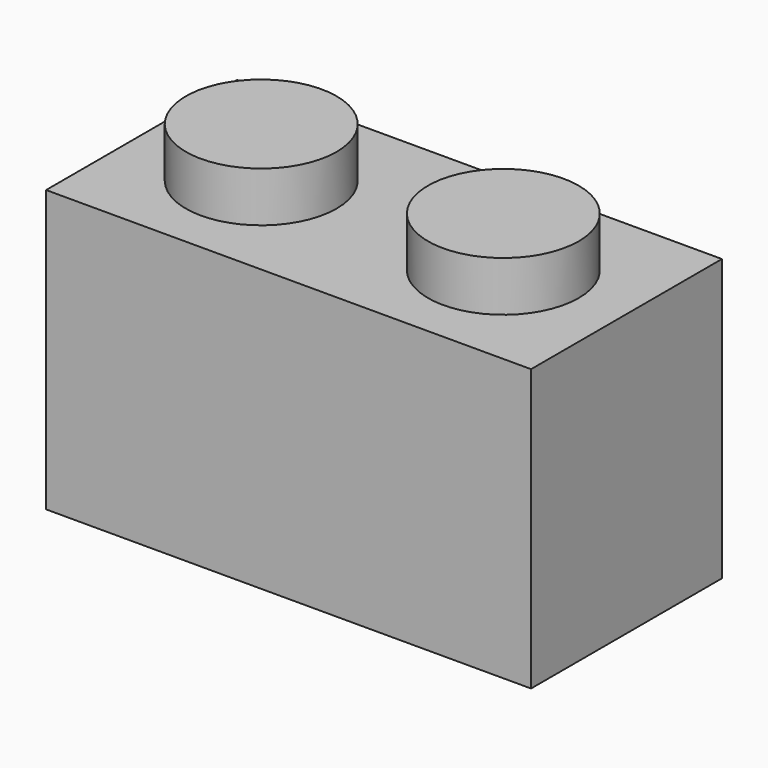
from build123d import *

# Parameters (mm, degrees)
F0_W      = 15.7734
F0_H      = 7.7597
F1_DEPTH  = 9.144
F2_R      = 2.4511
F3_DEPTH  = 1.6256
F5_W      = 13.0048
F5_H      = 4.953
F6_DEPTH  = 8.128
F7_R      = 1.5455831521
F8_DEPTH  = 8.128
F10_R     = 1.4732
F11_DEPTH = 8.128


# Not quite as in the source:
# - a feature names something its author has since deleted; it is built from what else it names


with BuildPart() as f1:
    # F0 (on Top) → F1 (new body)
    with BuildSketch(Plane.XY):
        with Locations((-0.3538653118, -22.1200450051)):
            Rectangle(F0_W, F0_H)
    extrude(amount=F1_DEPTH)

    # F2 (on face) → F3 (join)
    with BuildSketch(Plane.XY.offset(9.144)):
        with Locations((-4.2908653118, -22.1898950051)):
            Circle(F2_R)
        with Locations((3.5837523812, -22.1898950051)):
            Circle(F2_R)
    extrude(amount=F3_DEPTH)

    # F5 (on face) → F6 (cut)
    with BuildSketch(Plane(origin=(0, 0, 0), x_dir=(1, 0, 0), z_dir=(0, 0, -1))):
        with Locations((-0.3665653118, 22.1136950051)):
            Rectangle(F5_W, F5_H)
    extrude(amount=-F6_DEPTH, mode=Mode.SUBTRACT)

    # F10 (on Top) → F11 (join)
    with BuildSketch(Plane.XY):
        with Locations((-0.4554653118, -22.1390950051)):
            Circle(F10_R)
    extrude(amount=F11_DEPTH)


with BuildPart() as f8:
    # F7 (on face) → F8 (new body)
    with BuildSketch(Plane(origin=(0, 0, 0), x_dir=(1, 0, 0), z_dir=(0, 0, -1))):
        with Locations((-0.2611484639, 22.1479781572)):
            Circle(F7_R)
    extrude(amount=-F8_DEPTH)


solid = f1.part
